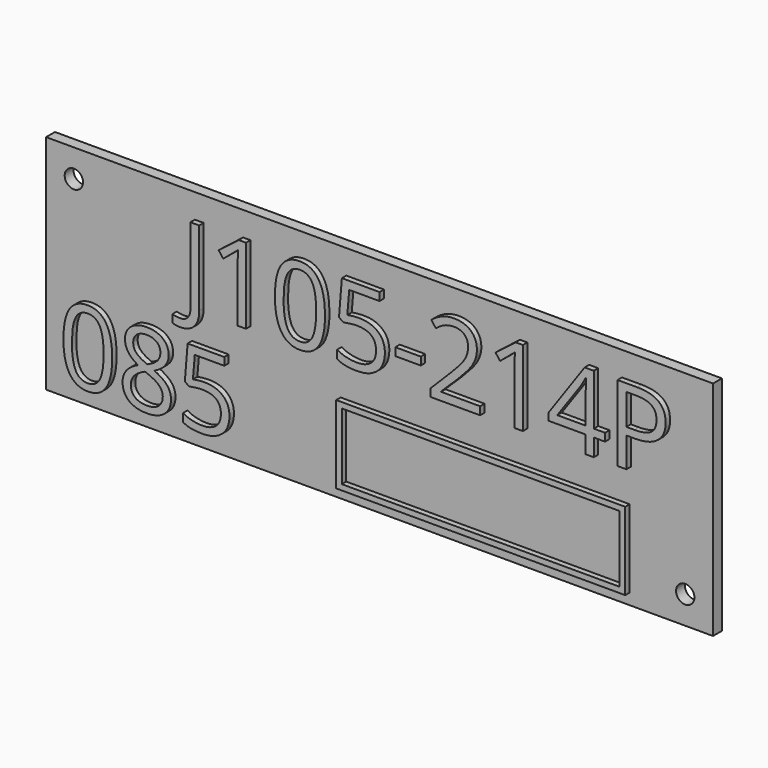
from build123d import *

# Parameters (mm, degrees)
F0_W         = 120
F0_H         = 40
F1_DEPTH     = 2
F3_D         = 3.3
F4_TEXT_SIZE = 19.0968768649
F5_DEPTH     = 1
F6_TEXT_SIZE = 18.5776487663
F7_DEPTH     = 1
F8_W         = 52
F8_H         = 14
F8_W_2       = 49.99999962
F8_H_2       = 11.99999962
F9_DEPTH     = 1


# Not quite as in the source:
# - Text() gives the source's letters only with a copy of the font that has no kerning and outlines rounded to 1/6400 em; it was checked with that copy


with BuildPart() as f1:
    # F0 (on Front) → F1 (new body)
    with BuildSketch(Plane.XZ):
        Rectangle(F0_W, F0_H)
    extrude(amount=F1_DEPTH)

    # F3 (through all)
    with Locations(Plane.XZ.offset(2)):
        with Locations((-55, 15), (55, -15)):
            Hole(F3_D / 2)

    # F4 (on face) → F5 (join)
    with BuildSketch(Plane.XZ.offset(2)):
        with Locations((-35, 2)):
            Text('J105-214P', F4_TEXT_SIZE, font='Open Sans', text_align=(TextAlign.LEFT, TextAlign.BOTTOM))
    extrude(amount=F5_DEPTH)

    # F6 (on face) → F7 (join)
    with BuildSketch(Plane.XZ.offset(2)):
        with Locations((-57, -17)):
            Text('085', F6_TEXT_SIZE, font='Open Sans', text_align=(TextAlign.LEFT, TextAlign.BOTTOM))
    extrude(amount=F7_DEPTH)

    # F8 (on face) → F9 (join)
    with BuildSketch(Plane.XZ.offset(2)):
        with Locations((19, -11)):
            Rectangle(F8_W, F8_H)
        with Locations((19, -11)):
            Rectangle(F8_W_2, F8_H_2, mode=Mode.SUBTRACT)
    extrude(amount=F9_DEPTH)


solid = f1.part
